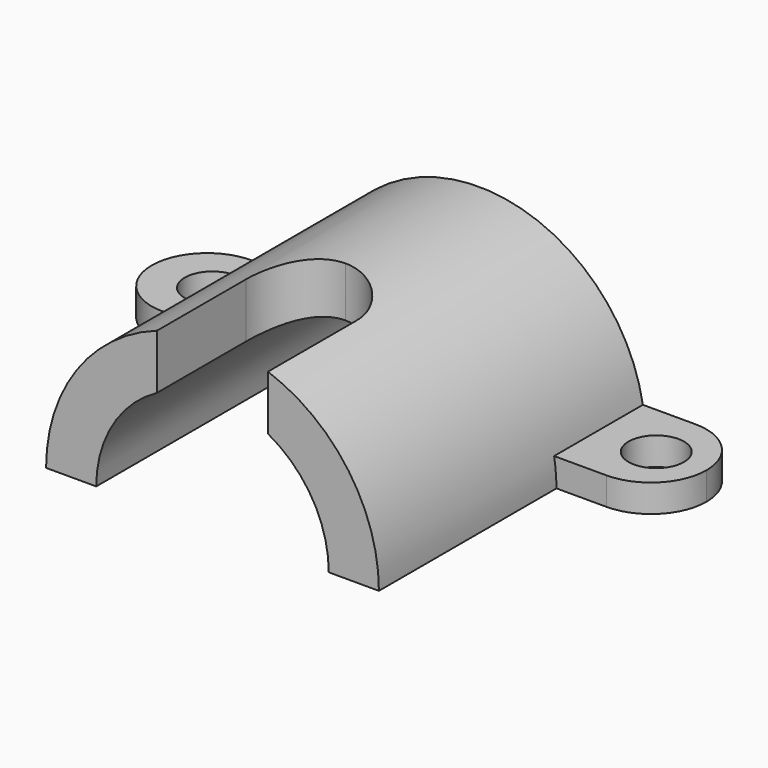
from build123d import *

# Parameters (mm, degrees)
F1_W      = 30
F1_H      = 60
F2_ANGLE  = 180
F3_W      = 100
F3_H      = 20
F4_DEPTH  = 5
F5_R      = 9.99999
F6_R      = 5
F7_DEPTH  = 30.001
F8_W      = 20
F8_H      = 30
F9_DEPTH  = 30.001
F10_R     = 9.999
F11_R     = 20.9596675634
F12_DEPTH = 60.0010001


# Not quite as in the source:
# - a fillet or chamfer is up to 0.001 mm smaller than in the source, because OpenCascade refuses the exact size


with BuildPart() as f2:
    # F1 (on Top) → F2 (revolve)
    with BuildSketch(Plane.XY):
        with Locations((15, 30)):
            Rectangle(F1_W, F1_H)
    revolve(axis=Axis((0, 30, 0), (0, -1, 0)), revolution_arc=F2_ANGLE)

    # F3 (on Top) → F4 (join)
    with BuildSketch(Plane.XY):
        with Locations((-0.9596675634, 50)):
            Rectangle(F3_W, F3_H)
    extrude(amount=F4_DEPTH)

    # F5 (radius 10 in the source; OpenCascade refuses exactly that, so slightly less here)
    f5_edges = [f2.edges().sort_by_distance(p)[0] for p in [
        (-50.959668, 60, 2.5),
        (-50.959668, 40, 2.5),
        (49.040332, 40, 2.5),
        (49.040332, 60, 2.5),
    ]]
    fillet(f5_edges, radius=F5_R)

    # F6 (on Top) → F7 (cut, through all)
    with BuildSketch(Plane.XY):
        with Locations((40, 50)):
            Circle(F6_R)
        with Locations((-40, 50)):
            Circle(F6_R)
    extrude(amount=F7_DEPTH, mode=Mode.SUBTRACT)

    # F8 (on Top) → F9 (cut, through all)
    with BuildSketch(Plane.XY):
        with Locations((0, 15)):
            Rectangle(F8_W, F8_H)
    extrude(amount=F9_DEPTH, mode=Mode.SUBTRACT)

    # F10 (radius 10 in the source; OpenCascade refuses exactly that, so slightly less here)
    f10_edges = [f2.edges().sort_by_distance(p)[0] for p in [
        (-10, 30, 14.142136),
        (10, 30, 14.142136),
    ]]
    fillet(f10_edges, radius=F10_R)

    # F11 (on face) → F12 (cut, through all)
    with BuildSketch(Plane(origin=(0, 60, 0), x_dir=(-1, 0, 0), z_dir=(0, 1, 0))):
        Circle(F11_R)
    extrude(amount=-F12_DEPTH, mode=Mode.SUBTRACT)


solid = f2.part
